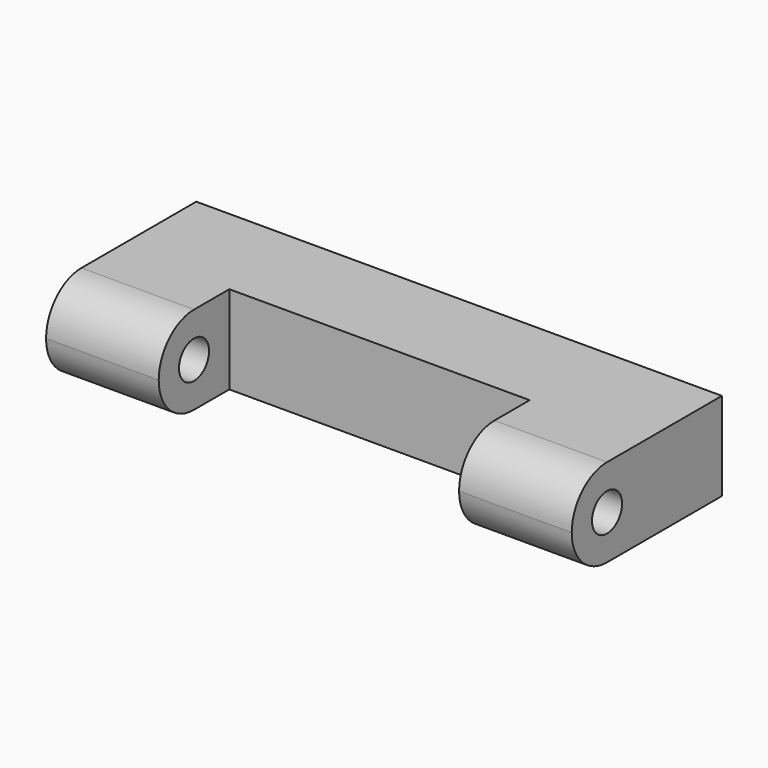
from build123d import *

# Parameters (mm, degrees)
F0_W     = 140
F0_H     = 23.5
F1_DEPTH = 50
F2_W     = 16
F2_H     = 16
F3_DEPTH = 15
F4_R     = 11.74999
F5_R     = 5
F6_DEPTH = 140
F8_DEPTH = 25


# Not quite as in the source:
# - a fillet or chamfer is up to 0.001 mm smaller than in the source, because OpenCascade refuses the exact size


with BuildPart() as f1:
    # F0 (on Front) → F1 (new body)
    with BuildSketch(Plane.XZ):
        with Locations((-8.7296748534, -19.8372076215)):
            Rectangle(F0_W, F0_H)
    extrude(amount=F1_DEPTH)

    # F2 (on face) → F3 (cut)
    with BuildSketch(Plane(origin=(0, 0, 0), x_dir=(-1, 0, 0), z_dir=(0, 1, 0))):
        with Locations((-41.2703251466, -21.5872076215)):
            Rectangle(F2_W, F2_H)
        with Locations((58.7296748534, -21.5872076215)):
            Rectangle(F2_W, F2_H)
    extrude(amount=-F3_DEPTH, mode=Mode.SUBTRACT)

    # F4 (radius 11.75 in the source; OpenCascade refuses exactly that, so slightly less here)
    f4_edges = [f1.edges().sort_by_distance(p)[0] for p in [
        (-8.729675, -50, -8.087208),
        (-8.729675, -50, -31.587208),
    ]]
    fillet(f4_edges, radius=F4_R)

    # F5 (on face) → F6 (cut, through all)
    with BuildSketch(Plane(origin=(-78.7296748534, 0, 0), x_dir=(0, -1, 0), z_dir=(-1, 0, 0))):
        with Locations((38.25, -19.8372076215)):
            Circle(F5_R)
    extrude(amount=-F6_DEPTH, mode=Mode.SUBTRACT)

    # F7 (on face) → F8 (cut)
    with BuildSketch(Plane(origin=(0, 0, -31.5872076215), x_dir=(1, 0, 0), z_dir=(0, 0, -1))):
        Polygon((31.2703251466, 51.5), (-8.7296748534, 51.5), (-48.7296748534, 51.5), (-48.7296748534, 26.5), (-8.7296748534, 26.5), (31.2703251466, 26.5), align=None)
    extrude(amount=-F8_DEPTH, mode=Mode.SUBTRACT)


solid = f1.part
